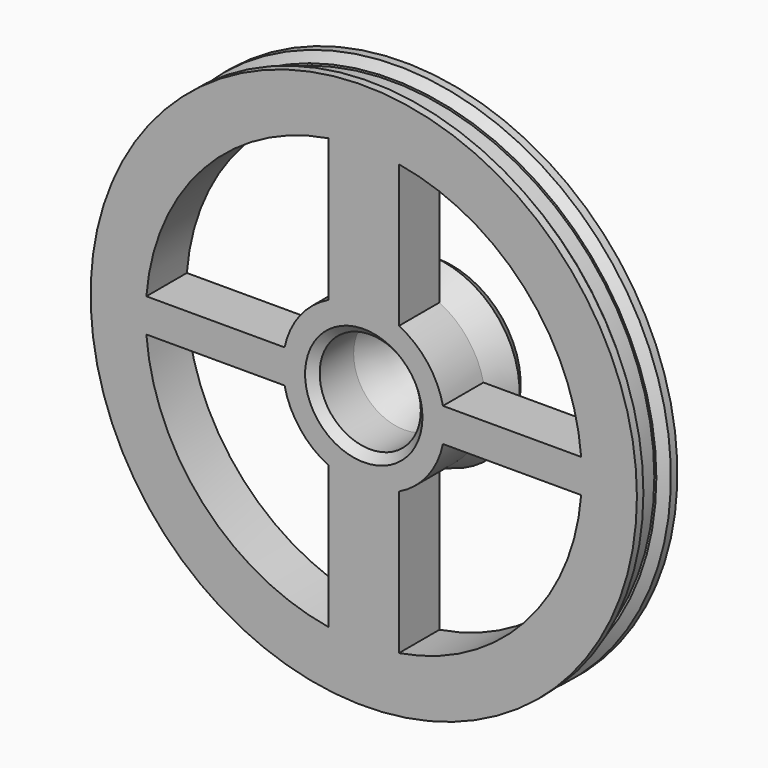
from build123d import *

# Parameters (mm, degrees)
F0_R     = 13
F0_R_2   = 2.5
F1_DEPTH = 2.5
F2_R     = 13.5
F2_R_2   = 10.9075922355
F3_DEPTH = 0.8
F4_R     = 13.5
F4_R_2   = 11.2490689916
F5_DEPTH = 0.8
F6_R     = 4
F6_R_2   = 2.5
F7_DEPTH = 2
F7_TAPER = -20


# Not quite as in the source:
# - a fillet or chamfer that OpenCascade refuses, or shapes differently, is made with other operations: its cross-section is extruded or revolved along the edge and cut away or added


with BuildPart() as f1:
    # F0 (on Front) → F1 (new body)
    with BuildSketch(Plane.XZ):
        Circle(F0_R)
        with BuildLine():
            ThreePointArc((-1.7385059182, -10.6337636412), (-7.9358324082, -7.2884769323), (-10.7429600727, -0.8295425725))
            Line((-10.7429600727, -0.8295425725), (-3.9130370712, -0.8295425725))
            ThreePointArc((-3.9130370712, -0.8295425725), (-3.1475751054, -2.468353896), (-1.7385059182, -3.6024432227))
            Line((-1.7385059182, -3.6024432227), (-1.7385059182, -10.6337636412))
        make_face(mode=Mode.SUBTRACT)
        with BuildLine():
            Line((3.9130370712, -0.8295425725), (10.7429600727, -0.8295425725))
            ThreePointArc((10.7429600727, -0.8295425725), (7.9358324082, -7.2884769323), (1.7385059182, -10.6337636412))
            Line((1.7385059182, -10.6337636412), (1.7385059182, -3.6024432227))
            ThreePointArc((1.7385059182, -3.6024432227), (3.1475751054, -2.468353896), (3.9130370712, -0.8295425725))
        make_face(mode=Mode.SUBTRACT)
        with BuildLine():
            ThreePointArc((-1.7385059182, 3.6024432227), (-3.1475751054, 2.468353896), (-3.9130370712, 0.8295425725))
            Line((-3.9130370712, 0.8295425725), (-10.7429600727, 0.8295425725))
            ThreePointArc((-10.7429600727, 0.8295425725), (-7.9358324082, 7.2884769323), (-1.7385059182, 10.6337636412))
            Line((-1.7385059182, 10.6337636412), (-1.7385059182, 3.6024432227))
        make_face(mode=Mode.SUBTRACT)
        Circle(F0_R_2, mode=Mode.SUBTRACT)
        with BuildLine():
            ThreePointArc((1.7385059182, 10.6337636412), (7.9358324082, 7.2884769323), (10.7429600727, 0.8295425725))
            Line((10.7429600727, 0.8295425725), (3.9130370712, 0.8295425725))
            ThreePointArc((3.9130370712, 0.8295425725), (3.1475751054, 2.468353896), (1.7385059182, 3.6024432227))
            Line((1.7385059182, 3.6024432227), (1.7385059182, 10.6337636412))
        make_face(mode=Mode.SUBTRACT)
    extrude(amount=F1_DEPTH)

    # F2 (on face) → F3 (join)
    with BuildSketch(Plane(origin=(0, 0, 0), x_dir=(-1, 0, 0), z_dir=(0, 1, 0))):
        Circle(F2_R)
        Circle(F2_R_2, mode=Mode.SUBTRACT)
    extrude(amount=-F3_DEPTH)

    # F4 (on face) → F5 (join)
    with BuildSketch(Plane.XZ.offset(2.5)):
        Circle(F4_R)
        Circle(F4_R_2, mode=Mode.SUBTRACT)
    extrude(amount=-F5_DEPTH)

    # F6 (on face) → F7 (join)
    with BuildSketch(Plane(origin=(0, 0, 0), x_dir=(-1, 0, 0), z_dir=(0, 1, 0))):
        Circle(F6_R)
        Circle(F6_R_2, mode=Mode.SUBTRACT)
    extrude(amount=F7_DEPTH, taper=F7_TAPER)

    # F8: chamfer of 0.4 on 4 edges, made by hand

    # F8_s1 → F8_t2 (revolve, cut)
    with BuildSketch(Plane.XY):
        Polygon((13.5, -2.1), (13.1, -1.7), (13.5, -1.7), align=None)
    revolve(axis=Axis((0, -1.7, 0), (0, -1, 0)), mode=Mode.SUBTRACT)

    # F8_s3 → F8_t4 (revolve, cut)
    with BuildSketch(Plane.XY):
        Polygon((-13.5, -0.4), (-13.1, -0.8), (-13.5, -0.8), align=None)
    revolve(axis=Axis((0, -0.8, 0), (0, 1, 0)), mode=Mode.SUBTRACT)

    # F8_s5 → F8_t6 (revolve, cut)
    with BuildSketch(Plane.XY):
        Polygon((2.9, -2.5), (2.5, -2.1), (2.5, -2.5), align=None)
    revolve(axis=Axis((0, -2.5, 0), (0, -1, 0)), mode=Mode.SUBTRACT)

    # F8_s7 → F8_t8 (revolve, cut)
    with BuildSketch(Plane.XY):
        Polygon((-4.5325583141, 1.4631919427), (-4.1566812658, 2), (-4.7279404685, 2), align=None)
    revolve(axis=Axis((0, 2, 0), (0, -1, 0)), mode=Mode.SUBTRACT)


solid = f1.part
